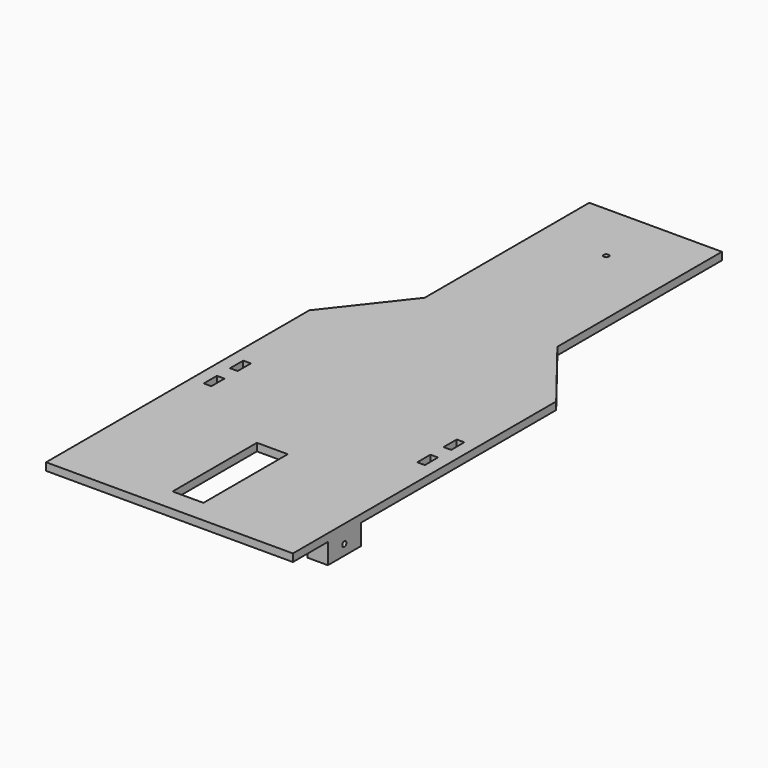
from build123d import *

# Parameters (mm, degrees)
F0_W     = 18.796
F0_H     = 40.64
F1_DEPTH = 18.796
F2_R     = 6.35
F3_DEPTH = 50.8
F4_W     = 101.6
F4_H     = 50.8
F4_R     = 6.35
F5_DEPTH = 50.8


# Not quite as in the source:
# - a feature names something its author has since deleted; it is built from what else it names


with BuildPart() as f1:
    # F0 (on Top) → F1 (new body)
    with BuildSketch(Plane.XY):
        Polygon((-163.8174757903, 706.2376797943), (-304.8, 526.2879983068), (-304.8, 30.9879983068), (-304.8, -286.5120016932), (304.8, -286.5120016932), (304.8, 30.9879983068), (304.8, 526.2879983068), (163.8174757903, 706.2376797943), (163.8174757903, 1214.2376797943), (-163.8174757903, 1214.2376797943), align=None)
        with Locations((-263.652, 180.8479983068)):
            Rectangle(F0_W, F0_H, mode=Mode.SUBTRACT)
        with Locations((-263.652, 262.1279983068)):
            Rectangle(F0_W, F0_H, mode=Mode.SUBTRACT)
        Polygon((38.1, 30.9879983068), (38.1, -229.3620016932), (-38.1, -229.3620016932), (-38.1, 30.9879983068), (0, 30.9879983068), align=None, mode=Mode.SUBTRACT)
        with Locations((263.652, 180.8479983068)):
            Rectangle(F0_W, F0_H, mode=Mode.SUBTRACT)
        with Locations((263.652, 262.1279983068)):
            Rectangle(F0_W, F0_H, mode=Mode.SUBTRACT)
        with BuildLine():
            ThreePointArc((0, 1055.4876797943), (-6.35, 1061.8376797943), (0, 1068.1876797943))
            ThreePointArc((0, 1068.1876797943), (4.4901280605, 1066.3278078548), (6.35, 1061.8376797943))
            ThreePointArc((6.35, 1061.8376797943), (4.4901280605, 1057.3475517337), (0, 1055.4876797943))
        make_face(mode=Mode.SUBTRACT)
    extrude(amount=F1_DEPTH)

    # F2 (on face) → F3 (join)
    with BuildSketch(Plane.YZ.offset(304.8)):
        Polygon((-127.7620016932, 0), (-178.5620016932, 0), (-178.5620016932, -50.8), (-127.7620016932, -50.8), (-76.9620016932, -50.8), (-76.9620016932, 0), align=None)
        with Locations((-127.7620016932, -25.4)):
            Circle(F2_R, mode=Mode.SUBTRACT)
    extrude(amount=-F3_DEPTH)

    # F4 (on face) → F5 (join)
    with BuildSketch(Plane(origin=(-304.8, 0, 0), x_dir=(0, -1, 0), z_dir=(-1, 0, 0))):
        with Locations((127.7626349211, -25.4)):
            Rectangle(F4_W, F4_H)
        with Locations((127.7626349211, -25.4)):
            Circle(F4_R, mode=Mode.SUBTRACT)
    extrude(amount=-F5_DEPTH)


solid = f1.part
